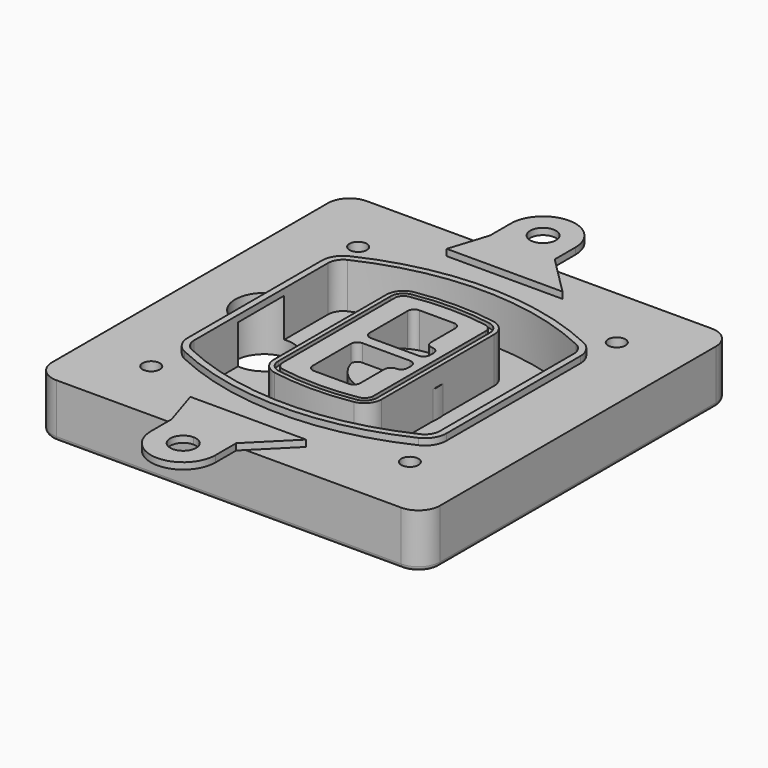
from build123d import *

# Parameters (mm, degrees)
F0_R      = 4
F1_DEPTH  = 25
F2_DEPTH  = 3
F3_DEPTH  = 18
F5_DEPTH  = 21
F6_DEPTH  = 2
F8_DEPTH  = 20
F9_DEPTH  = 16
F10_DEPTH = 25
F7_R      = 6
F7_R_2    = 4
F11_DEPTH = 6
F13_DEPTH = 9
F15_R     = 2
F17_DEPTH = 3


# Not quite as in the source:
# - a feature of the source that left no trace in its solid (it failed there, or was rolled back) is left out
# - a feature names something its author has since deleted; it is built from what else it names


with BuildPart() as f1:
    # F0 (on Top) → F1 (new body)
    with BuildSketch(Plane.XY):
        with BuildLine():
            ThreePointArc((-90, -80), (-87.0710678119, -87.0710678119), (-80, -90))
            Line((-80, -90), (80, -90))
            ThreePointArc((80, -90), (87.0710678119, -87.0710678119), (90, -80))
            Line((90, -80), (90, 80))
            ThreePointArc((90, 80), (87.0710678119, 87.0710678119), (80, 90))
            Line((80, 90), (-80, 90))
            ThreePointArc((-80, 90), (-87.0710678119, 87.0710678119), (-90, 80))
            Line((-90, 80), (-90, -80))
        make_face()
        with Locations((-60, -60)):
            Circle(F0_R, mode=Mode.SUBTRACT)
        with Locations((60, -60)):
            Circle(F0_R, mode=Mode.SUBTRACT)
        with Locations((-60, 60)):
            Circle(F0_R, mode=Mode.SUBTRACT)
        with BuildLine():
            ThreePointArc((-64, 38.8308515907), (-61.8195654598, 46.3340424013), (-55.9574468085, 51.5000594398))
            ThreePointArc((-55.9574468085, 51.5000594398), (0, 64), (55.9574468085, 51.5000594398))
            ThreePointArc((55.9574468085, 51.5000594398), (61.8195654598, 46.3340424013), (64, 38.8308515907))
            Line((64, 38.8308515907), (64, -38.8308515907))
            ThreePointArc((64, -38.8308515907), (61.8195654598, -46.3340424013), (55.9574468085, -51.5000594398))
            ThreePointArc((55.9574468085, -51.5000594398), (0, -64), (-55.9574468085, -51.5000594398))
            ThreePointArc((-55.9574468085, -51.5000594398), (-61.8195654598, -46.3340424013), (-64, -38.8308515907))
            Line((-64, -38.8308515907), (-64, 38.8308515907))
        make_face(mode=Mode.SUBTRACT)
        with Locations((60, 60)):
            Circle(F0_R, mode=Mode.SUBTRACT)
        with BuildLine():
            ThreePointArc((55.9574468085, 51.5000594398), (0, 64), (-55.9574468085, 51.5000594398))
            ThreePointArc((-55.9574468085, 51.5000594398), (-61.8195654598, 46.3340424013), (-64, 38.8308515907))
            Line((-64, 38.8308515907), (-64, -38.8308515907))
            ThreePointArc((-64, -38.8308515907), (-61.8195654598, -46.3340424013), (-55.9574468085, -51.5000594398))
            ThreePointArc((-55.9574468085, -51.5000594398), (0, -64), (55.9574468085, -51.5000594398))
            ThreePointArc((55.9574468085, -51.5000594398), (61.8195654598, -46.3340424013), (64, -38.8308515907))
            Line((64, -38.8308515907), (64, 38.8308515907))
            ThreePointArc((64, 38.8308515907), (61.8195654598, 46.3340424013), (55.9574468085, 51.5000594398))
        make_face()
        with BuildLine():
            Line((-60, -38.8308515907), (-60, 38.8308515907))
            ThreePointArc((-60, 38.8308515907), (-58.442546757, 44.1902735983), (-54.2553191489, 47.8802857686))
            ThreePointArc((-54.2553191489, 47.8802857686), (0, 60), (54.2553191489, 47.8802857686))
            ThreePointArc((54.2553191489, 47.8802857686), (58.442546757, 44.1902735983), (60, 38.8308515907))
            Line((60, 38.8308515907), (60, -38.8308515907))
            ThreePointArc((60, -38.8308515907), (58.442546757, -44.1902735983), (54.2553191489, -47.8802857686))
            ThreePointArc((54.2553191489, -47.8802857686), (0, -60), (-54.2553191489, -47.8802857686))
            ThreePointArc((-54.2553191489, -47.8802857686), (-58.442546757, -44.1902735983), (-60, -38.8308515907))
        make_face(mode=Mode.SUBTRACT)
        with BuildLine():
            ThreePointArc((-54.2553191489, 47.8802857686), (-58.442546757, 44.1902735983), (-60, 38.8308515907))
            Line((-60, 38.8308515907), (-60, -38.8308515907))
            ThreePointArc((-60, -38.8308515907), (-58.442546757, -44.1902735983), (-54.2553191489, -47.8802857686))
            ThreePointArc((-54.2553191489, -47.8802857686), (0, -60), (54.2553191489, -47.8802857686))
            ThreePointArc((54.2553191489, -47.8802857686), (58.442546757, -44.1902735983), (60, -38.8308515907))
            Line((60, -38.8308515907), (60, 38.8308515907))
            ThreePointArc((60, 38.8308515907), (58.442546757, 44.1902735983), (54.2553191489, 47.8802857686))
            ThreePointArc((54.2553191489, 47.8802857686), (0, 60), (-54.2553191489, 47.8802857686))
        make_face()
        with BuildLine():
            ThreePointArc((52.9787234043, 45.1654555152), (55.9097827299, 42.582446996), (57, 38.8308515907))
            Line((57, 38.8308515907), (57, -38.8308515907))
            ThreePointArc((57, -38.8308515907), (55.9097827299, -42.582446996), (52.9787234043, -45.1654555152))
            ThreePointArc((52.9787234043, -45.1654555152), (0, -57), (-52.9787234043, -45.1654555152))
            ThreePointArc((-52.9787234043, -45.1654555152), (-55.9097827299, -42.582446996), (-57, -38.8308515907))
            Line((-57, -38.8308515907), (-57, 38.8308515907))
            ThreePointArc((-57, 38.8308515907), (-55.9097827299, 42.582446996), (-52.9787234043, 45.1654555152))
            ThreePointArc((-52.9787234043, 45.1654555152), (0, 57), (52.9787234043, 45.1654555152))
        make_face(mode=Mode.SUBTRACT)
        with BuildLine():
            Line((57, -38.8308515907), (57, 38.8308515907))
            ThreePointArc((57, 38.8308515907), (55.9097827299, 42.582446996), (52.9787234043, 45.1654555152))
            ThreePointArc((52.9787234043, 45.1654555152), (0, 57), (-52.9787234043, 45.1654555152))
            ThreePointArc((-52.9787234043, 45.1654555152), (-55.9097827299, 42.582446996), (-57, 38.8308515907))
            Line((-57, 38.8308515907), (-57, -38.8308515907))
            ThreePointArc((-57, -38.8308515907), (-55.9097827299, -42.582446996), (-52.9787234043, -45.1654555152))
            ThreePointArc((-52.9787234043, -45.1654555152), (0, -57), (52.9787234043, -45.1654555152))
            ThreePointArc((52.9787234043, -45.1654555152), (55.9097827299, -42.582446996), (57, -38.8308515907))
        make_face()
    extrude(amount=-F1_DEPTH)

    # F0 (on Top) → F2 (join)
    with BuildSketch(Plane.XY):
        with BuildLine():
            ThreePointArc((-54.2553191489, 47.8802857686), (-58.442546757, 44.1902735983), (-60, 38.8308515907))
            Line((-60, 38.8308515907), (-60, -38.8308515907))
            ThreePointArc((-60, -38.8308515907), (-58.442546757, -44.1902735983), (-54.2553191489, -47.8802857686))
            ThreePointArc((-54.2553191489, -47.8802857686), (0, -60), (54.2553191489, -47.8802857686))
            ThreePointArc((54.2553191489, -47.8802857686), (58.442546757, -44.1902735983), (60, -38.8308515907))
            Line((60, -38.8308515907), (60, 38.8308515907))
            ThreePointArc((60, 38.8308515907), (58.442546757, 44.1902735983), (54.2553191489, 47.8802857686))
            ThreePointArc((54.2553191489, 47.8802857686), (0, 60), (-54.2553191489, 47.8802857686))
        make_face()
        with BuildLine():
            ThreePointArc((52.9787234043, 45.1654555152), (55.9097827299, 42.582446996), (57, 38.8308515907))
            Line((57, 38.8308515907), (57, -38.8308515907))
            ThreePointArc((57, -38.8308515907), (55.9097827299, -42.582446996), (52.9787234043, -45.1654555152))
            ThreePointArc((52.9787234043, -45.1654555152), (0, -57), (-52.9787234043, -45.1654555152))
            ThreePointArc((-52.9787234043, -45.1654555152), (-55.9097827299, -42.582446996), (-57, -38.8308515907))
            Line((-57, -38.8308515907), (-57, 38.8308515907))
            ThreePointArc((-57, 38.8308515907), (-55.9097827299, 42.582446996), (-52.9787234043, 45.1654555152))
            ThreePointArc((-52.9787234043, 45.1654555152), (0, 57), (52.9787234043, 45.1654555152))
        make_face(mode=Mode.SUBTRACT)
    extrude(amount=F2_DEPTH)

    # F0 (on Top) → F3 (cut)
    with BuildSketch(Plane.XY):
        with BuildLine():
            Line((57, -38.8308515907), (57, 38.8308515907))
            ThreePointArc((57, 38.8308515907), (55.9097827299, 42.582446996), (52.9787234043, 45.1654555152))
            ThreePointArc((52.9787234043, 45.1654555152), (0, 57), (-52.9787234043, 45.1654555152))
            ThreePointArc((-52.9787234043, 45.1654555152), (-55.9097827299, 42.582446996), (-57, 38.8308515907))
            Line((-57, 38.8308515907), (-57, -38.8308515907))
            ThreePointArc((-57, -38.8308515907), (-55.9097827299, -42.582446996), (-52.9787234043, -45.1654555152))
            ThreePointArc((-52.9787234043, -45.1654555152), (0, -57), (52.9787234043, -45.1654555152))
            ThreePointArc((52.9787234043, -45.1654555152), (55.9097827299, -42.582446996), (57, -38.8308515907))
        make_face()
    extrude(amount=-F3_DEPTH, mode=Mode.SUBTRACT)

    # F4 (on face) → F5 (join, through all)
    with BuildSketch(Plane.XY.offset(3)):
        with BuildLine():
            ThreePointArc((-25, -32.5662280692), (-23.1122504785, -37.7276614059), (-18.3399014778, -40.4532214146))
            ThreePointArc((-18.3399014778, -40.4532214146), (0, -42), (18.3399014778, -40.4532214146))
            ThreePointArc((18.3399014778, -40.4532214146), (23.1122504785, -37.7276614059), (25, -32.5662280692))
            Line((25, -32.5662280692), (25, 32.5662280692))
            ThreePointArc((25, 32.5662280692), (23.1122504785, 37.7276614059), (18.3399014778, 40.4532214146))
            ThreePointArc((18.3399014778, 40.4532214146), (0, 42), (-18.3399014778, 40.4532214146))
            ThreePointArc((-18.3399014778, 40.4532214146), (-23.1122504785, 37.7276614059), (-25, 32.5662280692))
            Line((-25, 32.5662280692), (-25, -32.5662280692))
        make_face()
        with BuildLine():
            ThreePointArc((18.0049261084, 38.4814730782), (21.5841878588, 36.4373030717), (23, 32.5662280692))
            Line((23, 32.5662280692), (23, -32.5662280692))
            ThreePointArc((23, -32.5662280692), (21.5841878588, -36.4373030717), (18.0049261084, -38.4814730782))
            ThreePointArc((18.0049261084, -38.4814730782), (0, -40), (-18.0049261084, -38.4814730782))
            ThreePointArc((-18.0049261084, -38.4814730782), (-21.5841878588, -36.4373030717), (-23, -32.5662280692))
            Line((-23, -32.5662280692), (-23, 32.5662280692))
            ThreePointArc((-23, 32.5662280692), (-21.5841878588, 36.4373030717), (-18.0049261084, 38.4814730782))
            ThreePointArc((-18.0049261084, 38.4814730782), (0, 40), (18.0049261084, 38.4814730782))
        make_face(mode=Mode.SUBTRACT)
        with BuildLine():
            Line((23, -32.5662280692), (23, 32.5662280692))
            ThreePointArc((23, 32.5662280692), (21.5841878588, 36.4373030717), (18.0049261084, 38.4814730782))
            ThreePointArc((18.0049261084, 38.4814730782), (0, 40), (-18.0049261084, 38.4814730782))
            ThreePointArc((-18.0049261084, 38.4814730782), (-21.5841878588, 36.4373030717), (-23, 32.5662280692))
            Line((-23, 32.5662280692), (-23, -32.5662280692))
            ThreePointArc((-23, -32.5662280692), (-21.5841878588, -36.4373030717), (-18.0049261084, -38.4814730782))
            ThreePointArc((-18.0049261084, -38.4814730782), (0, -40), (18.0049261084, -38.4814730782))
            ThreePointArc((18.0049261084, -38.4814730782), (21.5841878588, -36.4373030717), (23, -32.5662280692))
        make_face()
        with BuildLine():
            ThreePointArc((17.6699507389, 36.5097247419), (20.0561252392, 35.1469447375), (21, 32.5662280692))
            Line((21, 32.5662280692), (21, -32.5662280692))
            ThreePointArc((21, -32.5662280692), (20.0561252392, -35.1469447375), (17.6699507389, -36.5097247419))
            ThreePointArc((17.6699507389, -36.5097247419), (0, -38), (-17.6699507389, -36.5097247419))
            ThreePointArc((-17.6699507389, -36.5097247419), (-20.0561252392, -35.1469447375), (-21, -32.5662280692))
            Line((-21, -32.5662280692), (-21, 32.5662280692))
            ThreePointArc((-21, 32.5662280692), (-20.0561252392, 35.1469447375), (-17.6699507389, 36.5097247419))
            ThreePointArc((-17.6699507389, 36.5097247419), (0, 38), (17.6699507389, 36.5097247419))
        make_face(mode=Mode.SUBTRACT)
        with BuildLine():
            Line((21, -32.5662280692), (21, 32.5662280692))
            ThreePointArc((21, 32.5662280692), (20.0561252392, 35.1469447375), (17.6699507389, 36.5097247419))
            ThreePointArc((17.6699507389, 36.5097247419), (0, 38), (-17.6699507389, 36.5097247419))
            ThreePointArc((-17.6699507389, 36.5097247419), (-20.0561252392, 35.1469447375), (-21, 32.5662280692))
            Line((-21, 32.5662280692), (-21, -32.5662280692))
            ThreePointArc((-21, -32.5662280692), (-20.0561252392, -35.1469447375), (-17.6699507389, -36.5097247419))
            ThreePointArc((-17.6699507389, -36.5097247419), (0, -38), (17.6699507389, -36.5097247419))
            ThreePointArc((17.6699507389, -36.5097247419), (20.0561252392, -35.1469447375), (21, -32.5662280692))
        make_face()
        with BuildLine():
            Line((-8, -2.5), (14, -2.5))
            ThreePointArc((14, -2.5), (16.1213203436, -3.3786796564), (17, -5.5))
            Line((17, -5.5), (17, -7.5))
            ThreePointArc((17, -7.5), (16.1213203436, -9.6213203436), (14, -10.5))
            ThreePointArc((14, -10.5), (11.8786796564, -11.3786796564), (11, -13.5))
            Line((11, -13.5), (11, -27.5))
            ThreePointArc((11, -27.5), (10.1213203436, -29.6213203436), (8, -30.5))
            Line((8, -30.5), (-8, -30.5))
            ThreePointArc((-8, -30.5), (-10.1213203436, -29.6213203436), (-11, -27.5))
            Line((-11, -27.5), (-11, -5.5))
            ThreePointArc((-11, -5.5), (-10.1213203436, -3.3786796564), (-8, -2.5))
        make_face(mode=Mode.SUBTRACT)
        with BuildLine():
            ThreePointArc((-8, 2.5), (-10.1213203436, 3.3786796564), (-11, 5.5))
            Line((-11, 5.5), (-11, 27.5))
            ThreePointArc((-11, 27.5), (-10.1213203436, 29.6213203436), (-8, 30.5))
            Line((-8, 30.5), (8, 30.5))
            ThreePointArc((8, 30.5), (10.1213203436, 29.6213203436), (11, 27.5))
            Line((11, 27.5), (11, 13.5))
            ThreePointArc((11, 13.5), (11.8786796564, 11.3786796564), (14, 10.5))
            ThreePointArc((14, 10.5), (16.1213203436, 9.6213203436), (17, 7.5))
            Line((17, 7.5), (17, 5.5))
            ThreePointArc((17, 5.5), (16.1213203436, 3.3786796564), (14, 2.5))
            Line((14, 2.5), (-8, 2.5))
        make_face(mode=Mode.SUBTRACT)
    extrude(amount=-F5_DEPTH)

    # F4 (on face) → F6 (cut)
    with BuildSketch(Plane.XY.offset(3)):
        with BuildLine():
            Line((23, -32.5662280692), (23, 32.5662280692))
            ThreePointArc((23, 32.5662280692), (21.5841878588, 36.4373030717), (18.0049261084, 38.4814730782))
            ThreePointArc((18.0049261084, 38.4814730782), (0, 40), (-18.0049261084, 38.4814730782))
            ThreePointArc((-18.0049261084, 38.4814730782), (-21.5841878588, 36.4373030717), (-23, 32.5662280692))
            Line((-23, 32.5662280692), (-23, -32.5662280692))
            ThreePointArc((-23, -32.5662280692), (-21.5841878588, -36.4373030717), (-18.0049261084, -38.4814730782))
            ThreePointArc((-18.0049261084, -38.4814730782), (0, -40), (18.0049261084, -38.4814730782))
            ThreePointArc((18.0049261084, -38.4814730782), (21.5841878588, -36.4373030717), (23, -32.5662280692))
        make_face()
        with BuildLine():
            ThreePointArc((17.6699507389, 36.5097247419), (20.0561252392, 35.1469447375), (21, 32.5662280692))
            Line((21, 32.5662280692), (21, -32.5662280692))
            ThreePointArc((21, -32.5662280692), (20.0561252392, -35.1469447375), (17.6699507389, -36.5097247419))
            ThreePointArc((17.6699507389, -36.5097247419), (0, -38), (-17.6699507389, -36.5097247419))
            ThreePointArc((-17.6699507389, -36.5097247419), (-20.0561252392, -35.1469447375), (-21, -32.5662280692))
            Line((-21, -32.5662280692), (-21, 32.5662280692))
            ThreePointArc((-21, 32.5662280692), (-20.0561252392, 35.1469447375), (-17.6699507389, 36.5097247419))
            ThreePointArc((-17.6699507389, 36.5097247419), (0, 38), (17.6699507389, 36.5097247419))
        make_face(mode=Mode.SUBTRACT)
    extrude(amount=-F6_DEPTH, mode=Mode.SUBTRACT)

    # F7 (on face) → F8 (join)
    with BuildSketch(Plane(origin=(0, 0, -25), x_dir=(1, 0, 0), z_dir=(0, 0, -1))):
        with BuildLine():
            ThreePointArc((-6.71157564, 0), (6.7567035675, 13.4682792075), (20.224982775, 0))
            Line((20.224982775, 0), (25.224982775, 0))
            ThreePointArc((25.224982775, 0), (6.7567035675, 18.4682792075), (-11.71157564, 0))
            Line((-11.71157564, 0), (-6.71157564, 0))
        make_face()
        with BuildLine():
            Line((-6.71157564, 0), (20.224982775, 0))
            ThreePointArc((20.224982775, 0), (6.7567035675, 13.4682792075), (-6.71157564, 0))
        make_face()
        with BuildLine():
            ThreePointArc((-6.71157564, 0), (6.7567035675, -13.4682792075), (20.224982775, 0))
            Line((20.224982775, 0), (-6.71157564, 0))
        make_face()
        with BuildLine():
            Line((25.224982775, 0), (20.224982775, 0))
            ThreePointArc((20.224982775, 0), (6.7567035675, -13.4682792075), (-6.71157564, 0))
            Line((-6.71157564, 0), (-11.71157564, 0))
            ThreePointArc((-11.71157564, 0), (6.7567035675, -18.4682792075), (25.224982775, 0))
        make_face()
    extrude(amount=-F8_DEPTH)

    # F7 (on face) → F9 (cut)
    with BuildSketch(Plane(origin=(0, 0, -25), x_dir=(1, 0, 0), z_dir=(0, 0, -1))):
        with BuildLine():
            Line((-6.71157564, 0), (20.224982775, 0))
            ThreePointArc((20.224982775, 0), (6.7567035675, 13.4682792075), (-6.71157564, 0))
        make_face()
        with BuildLine():
            ThreePointArc((-6.71157564, 0), (6.7567035675, -13.4682792075), (20.224982775, 0))
            Line((20.224982775, 0), (-6.71157564, 0))
        make_face()
    extrude(amount=-F9_DEPTH, mode=Mode.SUBTRACT)

    # F7 (on face) → F10 (cut)
    with BuildSketch(Plane(origin=(0, 0, -25), x_dir=(1, 0, 0), z_dir=(0, 0, -1))):
        with BuildLine():
            Line((-69.0318229325, 0), (-42.0952645175, 0))
            ThreePointArc((-42.0952645175, 0), (-55.563543725, 13.4682792075), (-69.0318229325, 0))
        make_face()
        with BuildLine():
            ThreePointArc((-69.0318229325, 0), (-55.563543725, -13.4682792075), (-42.0952645175, 0))
            Line((-42.0952645175, 0), (-69.0318229325, 0))
        make_face()
    extrude(amount=-F10_DEPTH, mode=Mode.SUBTRACT)

    # F7 (on face) → F11 (cut)
    with BuildSketch(Plane(origin=(0, 0, -25), x_dir=(1, 0, 0), z_dir=(0, 0, -1))):
        with Locations((60, -60)):
            Circle(F7_R)
        with Locations((60, -60)):
            Circle(F7_R_2, mode=Mode.SUBTRACT)
        with Locations((-60, -60)):
            Circle(F7_R)
        with Locations((-60, -60)):
            Circle(F7_R_2, mode=Mode.SUBTRACT)
        with Locations((-60, 60)):
            Circle(F7_R)
        with Locations((-60, 60)):
            Circle(F7_R_2, mode=Mode.SUBTRACT)
        with Locations((60, 60)):
            Circle(F7_R)
        with Locations((60, 60)):
            Circle(F7_R_2, mode=Mode.SUBTRACT)
    extrude(amount=-F11_DEPTH, mode=Mode.SUBTRACT)

    # F12 (on face) → F13 (cut, through all)
    with BuildSketch(Plane(origin=(0, 0, -9), x_dir=(1, 0, 0), z_dir=(0, 0, -1))):
        with BuildLine():
            ThreePointArc((20.224982775, 0), (20.1663399806, 1.2554664788), (19.9909222755, 2.5))
            Line((19.9909222755, 2.5), (14, 2.5))
            ThreePointArc((14, 2.5), (16.1213203436, 3.3786796564), (17, 5.5))
            Line((17, 5.5), (17, 7.5))
            ThreePointArc((17, 7.5), (16.1213203436, 9.6213203436), (14, 10.5))
            ThreePointArc((14, 10.5), (12.1627255951, 11.1284134507), (11.0951631559, 12.750384826))
            ThreePointArc((11.0951631559, 12.750384826), (11.0476113807, 12.7664660322), (11, 12.7823698976))
            Line((11, 12.7823698976), (11, -12.7823698976))
            ThreePointArc((11, -12.7823698976), (11.0476113807, -12.7664660322), (11.0951631559, -12.750384826))
            ThreePointArc((11.0951631559, -12.750384826), (12.1627255951, -11.1284134507), (14, -10.5))
            ThreePointArc((14, -10.5), (16.1213203436, -9.6213203436), (17, -7.5))
            Line((17, -7.5), (17, -5.5))
            ThreePointArc((17, -5.5), (16.1213203436, -3.3786796564), (14, -2.5))
            Line((14, -2.5), (19.9909222755, -2.5))
            ThreePointArc((19.9909222755, -2.5), (20.1663399806, -1.2554664788), (20.224982775, 0))
        make_face()
    extrude(amount=F13_DEPTH, mode=Mode.SUBTRACT)

    # F15
    f15_edges = [f1.edges().sort_by_distance(p)[0] for p in [
        (0, -90, -25),
        (-87.071068, -87.071068, -25),
        (-90, 0, -25),
        (-87.071068, 87.071068, -25),
        (87.071068, -87.071068, -25),
        (0, 90, -25),
        (90, 0, -25),
        (87.071068, 87.071068, -25),
    ]]
    fillet(f15_edges, radius=F15_R)


with BuildPart() as f17:
    # F16 (on Top) → F17 (new body, through all)
    with BuildSketch(Plane.XY):
        with BuildLine():
            Line((-24.6755290329, 92.3539854884), (-30.3919422144, 74.3539854884))
            Line((-30.3919422144, 74.3539854884), (-9.6755290329, 74.3539854884))
            Line((-9.6755290329, 74.3539854884), (23.3244709671, 74.3539854884))
            Line((23.3244709671, 74.3539854884), (5.3244709671, 92.3539854884))
            Line((5.3244709671, 92.3539854884), (5.3244709671, 104.3539854884))
            ThreePointArc((5.3244709671, 104.3539854884), (-9.6755290329, 119.3539854884), (-24.6755290329, 104.3539854884))
            Line((-24.6755290329, 104.3539854884), (-24.6755290329, 92.3539854884))
        make_face()
        with BuildLine():
            ThreePointArc((-3.6755290329, 104.3539854884), (-5.4328883458, 100.1113448013), (-9.6755290329, 98.3539854884))
            ThreePointArc((-9.6755290329, 98.3539854884), (-13.9181697201, 108.5966261755), (-3.6755290329, 104.3539854884))
        make_face(mode=Mode.SUBTRACT)
    extrude(amount=F17_DEPTH)


with BuildPart() as f17b:
    # F16 (on Top) → F17, piece 2 (new body, through all)
    with BuildSketch(Plane.XY):
        with BuildLine():
            ThreePointArc((-24.6755290329, -104.3539854884), (-9.6755290329, -119.3539854884), (5.3244709671, -104.3539854884))
            Line((5.3244709671, -104.3539854884), (5.3244709671, -92.3539854884))
            Line((5.3244709671, -92.3539854884), (23.3244709671, -74.3539854884))
            Line((23.3244709671, -74.3539854884), (-9.6755290329, -74.3539854884))
            Line((-9.6755290329, -74.3539854884), (-30.3919422144, -74.3539854884))
            Line((-30.3919422144, -74.3539854884), (-24.6755290329, -92.3539854884))
            Line((-24.6755290329, -92.3539854884), (-24.6755290329, -104.3539854884))
        make_face()
        with BuildLine():
            ThreePointArc((-3.6755290329, -104.3539854884), (-13.9181697201, -108.5966261755), (-9.6755290329, -98.3539854884))
            ThreePointArc((-9.6755290329, -98.3539854884), (-5.4328883458, -100.1113448013), (-3.6755290329, -104.3539854884))
        make_face(mode=Mode.SUBTRACT)
    extrude(amount=F17_DEPTH)


solid = Compound([f1.part, f17.part, f17b.part])
